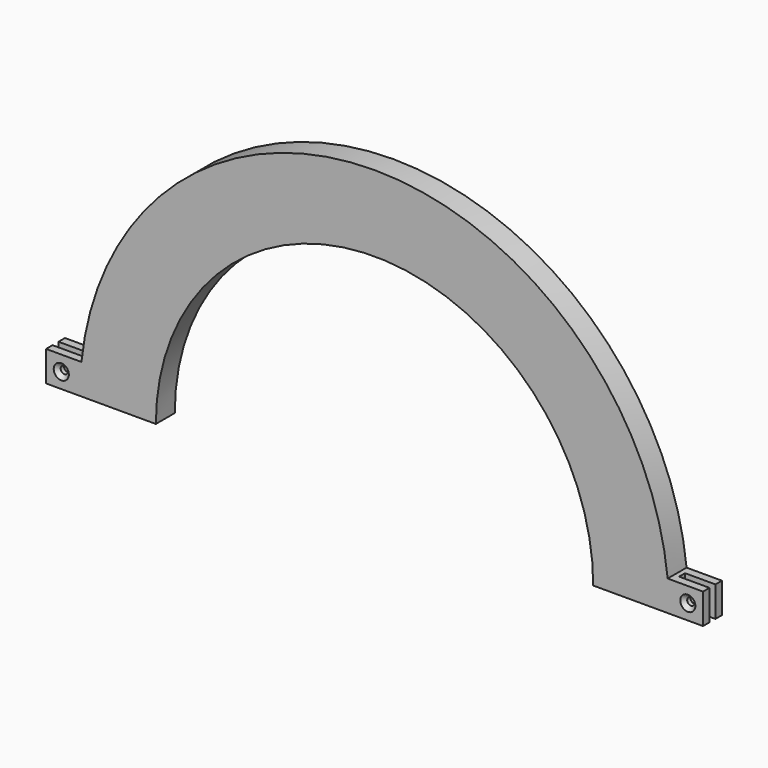
from build123d import *

# Parameters (mm, degrees)
F1_DEPTH       = 7
F2_DEPTH       = 6
F3_W           = 4.4
F3_H           = 18
F4_DEPTH       = 18
F6_D           = 4.4
F6_DEPTH       = 5
F6_CSINK_D     = 8.96
F6_CSINK_ANGLE = 90
F6_TIP         = 1.3218933619
F8_DEPTH       = 2.6
F9_R           = 2.2
F10_DEPTH      = 2.3


# Not quite as in the source:
# - a pattern or mirror of a feature is missing from the dataset's text; its kind, count and spacing are read off the source's solid


with BuildPart() as f1:
    # F0 (on Front) → F1 (new body, symmetric)
    with BuildSketch(Plane.XZ):
        with BuildLine():
            Line((129.5, 0), (174.5, 0))
            ThreePointArc((174.5, 0), (174.2671322418, 9.0120264206), (173.5691504848, 18))
            ThreePointArc((173.5691504848, 18), (0, 174.5), (-173.5691504848, 18))
            ThreePointArc((-173.5691504848, 18), (-174.2671322418, 9.0120264206), (-174.5, 0))
            Line((-174.5, 0), (-129.5, 0))
            ThreePointArc((-129.5, 0), (0, 129.5), (129.5, 0))
        make_face()
        with BuildLine():
            ThreePointArc((173.5691504848, 18), (174.2671322418, 9.0120264206), (174.5, 0))
            Line((174.5, 0), (194.5, 0))
            Line((194.5, 0), (194.5, 18))
            Line((194.5, 18), (173.5691504848, 18))
        make_face()
        with BuildLine():
            ThreePointArc((-174.5, 0), (-174.2671322418, 9.0120264206), (-173.5691504848, 18))
            Line((-173.5691504848, 18), (-194.5, 18))
            Line((-194.5, 18), (-194.5, 0))
            Line((-194.5, 0), (-174.5, 0))
        make_face()
    extrude(amount=F1_DEPTH, both=True)

    # F0 (on Front) → F2 (join, symmetric)
    with BuildSketch(Plane.XZ):
        with BuildLine():
            Line((129.5, 0), (174.5, 0))
            ThreePointArc((174.5, 0), (174.2671322418, 9.0120264206), (173.5691504848, 18))
            ThreePointArc((173.5691504848, 18), (0, 174.5), (-173.5691504848, 18))
            ThreePointArc((-173.5691504848, 18), (-174.2671322418, 9.0120264206), (-174.5, 0))
            Line((-174.5, 0), (-129.5, 0))
            ThreePointArc((-129.5, 0), (0, 129.5), (129.5, 0))
        make_face()
        with BuildLine():
            ThreePointArc((173.5691504848, 18), (174.2671322418, 9.0120264206), (174.5, 0))
            Line((174.5, 0), (194.5, 0))
            Line((194.5, 0), (194.5, 18))
            Line((194.5, 18), (173.5691504848, 18))
        make_face()
        with BuildLine():
            ThreePointArc((-174.5, 0), (-174.2671322418, 9.0120264206), (-173.5691504848, 18))
            Line((-173.5691504848, 18), (-194.5, 18))
            Line((-194.5, 18), (-194.5, 0))
            Line((-194.5, 0), (-174.5, 0))
        make_face()
    extrude(amount=F2_DEPTH, both=True)

    # F3 (on face) → F4 (cut)
    with BuildSketch(Plane.YZ.offset(194.5)):
        with Locations((0, 9)):
            Rectangle(F3_W, F3_H)
    f4 = extrude(amount=-F4_DEPTH, mode=Mode.SUBTRACT)

    # F4_copies: F4 across plane
    add(f4.mirror(Plane(origin=(0, 0, 0), x_dir=(0, 0, -1), z_dir=(-1, 0, 0))), mode=Mode.SUBTRACT)

    # F6
    with Locations(Plane.XZ.offset(7)):
        with Locations((185.5, 9)):
            f6 = CounterSinkHole(F6_D / 2, F6_CSINK_D / 2, depth=F6_DEPTH, counter_sink_angle=F6_CSINK_ANGLE)
            with Locations((0, 0, -(F6_DEPTH + F6_TIP / 2))):  # 118° drill point
                Cone(0, F6_D / 2, F6_TIP, mode=Mode.SUBTRACT)

    # F6_copies: F6 across plane
    add(f6.mirror(Plane(origin=(0, 0, 0), x_dir=(0, 0, -1), z_dir=(-1, 0, 0))), mode=Mode.SUBTRACT)

    # F7 (on face) → F8 (cut)
    with BuildSketch(Plane(origin=(0, 7, 0), x_dir=(-1, 0, 0), z_dir=(0, 1, 0))):
        Polygon((-189, 11.0207259422), (-189, 6.9792740578), (-185.5, 4.9585481157), (-182, 6.9792740578), (-182, 11.0207259422), (-185.5, 13.0414518843), align=None)
    f8 = extrude(amount=-F8_DEPTH, mode=Mode.SUBTRACT)

    # F8_copies: F8 across plane
    add(f8.mirror(Plane(origin=(0, 0, 0), x_dir=(0, 0, -1), z_dir=(-1, 0, 0))), mode=Mode.SUBTRACT)

    # F9 (on face) → F10 (cut)
    with BuildSketch(Plane(origin=(0, 4.4, 0), x_dir=(-1, 0, 0), z_dir=(0, 1, 0))):
        with Locations((-185.5, 9)):
            Circle(F9_R)
    f10 = extrude(amount=-F10_DEPTH, mode=Mode.SUBTRACT)

    # F10_copies: F10 across plane
    add(f10.mirror(Plane(origin=(0, 0, 0), x_dir=(0, 0, -1), z_dir=(-1, 0, 0))), mode=Mode.SUBTRACT)


solid = f1.part
